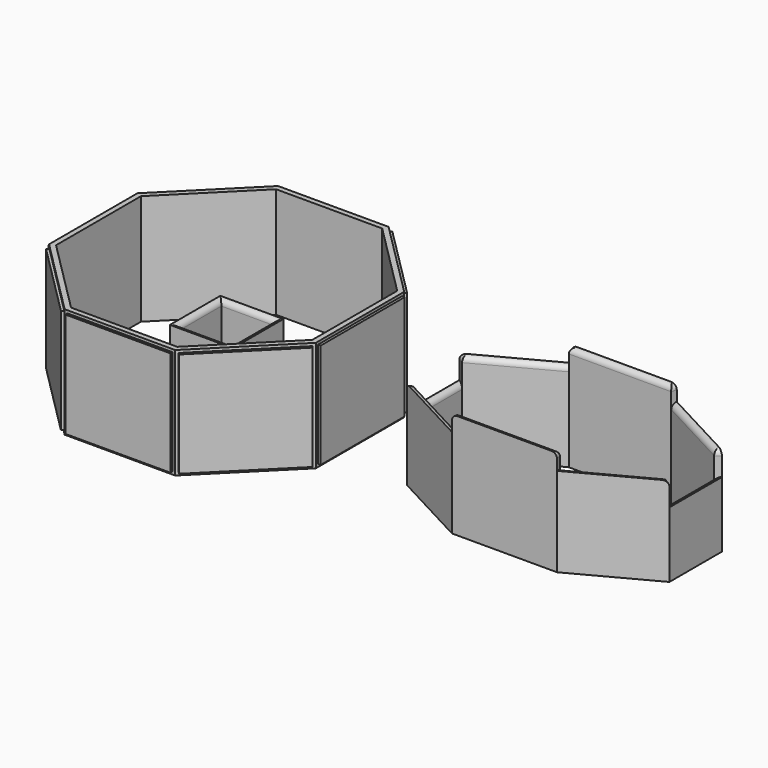
from build123d import *

# Parameters (mm, degrees)
F1_DEPTH  = 42.0840916
F2_W      = 24
F2_H      = 24
F2_W_2    = 20
F2_H_2    = 20
F3_DEPTH  = 24
F4_W      = 40
F4_H      = 40
F5_DEPTH  = 1
F7_COUNT  = 8
F9_DEPTH  = 25
F10_DEPTH = 40
F11_DEPTH = 34
F12_R     = 1.99999
F13_R     = 1.99999


# Not quite as in the source:
# - a fillet or chamfer is up to 0.001 mm smaller than in the source, because OpenCascade refuses the exact size


with BuildPart() as f1:
    # F0 (on Top) → F1 (new body)
    with BuildSketch(Plane.XY):
        Polygon((-50.8, 21.0420489686), (-50.8, -21.0420489686), (-21.0420489686, -50.8), (21.0420489686, -50.8), (50.8, -21.0420489686), (50.8, 21.0420489686), (21.0420489686, 50.8), (-21.0420489686, 50.8), align=None)
        Polygon((-20.2136218438, -48.8), (-48.8, -20.2136218438), (-48.8, 20.2136218438), (-20.2136218438, 48.8), (20.2136218438, 48.8), (48.8, 20.2136218438), (48.8, -20.2136218438), (20.2136218438, -48.8), align=None, mode=Mode.SUBTRACT)
    extrude(amount=F1_DEPTH)


with BuildPart() as f3:
    # F2 (on Top) → F3 (new body)
    with BuildSketch(Plane.XY):
        Rectangle(F2_W, F2_H)
        Rectangle(F2_W_2, F2_H_2, mode=Mode.SUBTRACT)
    extrude(amount=F3_DEPTH)

    # F13 (radius 2 in the source; OpenCascade refuses exactly that, so slightly less here)
    f13_edges = [f3.edges().sort_by_distance(p)[0] for p in [
        (0, 10, 24),
        (-10, 0, 24),
        (10, 0, 24),
        (0, -10, 24),
    ]]
    fillet(f13_edges, radius=F13_R)


with BuildPart() as f5:
    # F4 (on face) → F5 (new body, symmetric)
    with BuildSketch(Plane(origin=(0, 50.8, 0), x_dir=(-1, 0, 0), z_dir=(0, 1, 0))):
        with Locations((0, 21.0420458)):
            Rectangle(F4_W, F4_H)
    extrude(amount=F5_DEPTH, both=True)


with BuildPart() as f7_1:
    # F7: instance of F5
    add(f5.part.rotate(Axis((0, 0, 32.1497656405), (0, 0, 1)), 1 * 360 / F7_COUNT))


with BuildPart() as f7_2:
    # F7: instance of F5
    add(f5.part.rotate(Axis((0, 0, 32.1497656405), (0, 0, 1)), 2 * 360 / F7_COUNT))


with BuildPart() as f7_3:
    # F7: instance of F5
    add(f5.part.rotate(Axis((0, 0, 32.1497656405), (0, 0, 1)), 3 * 360 / F7_COUNT))


with BuildPart() as f7_4:
    # F7: instance of F5
    add(f5.part.rotate(Axis((0, 0, 32.1497656405), (0, 0, 1)), 4 * 360 / F7_COUNT))


with BuildPart() as f7_5:
    # F7: instance of F5
    add(f5.part.rotate(Axis((0, 0, 32.1497656405), (0, 0, 1)), 5 * 360 / F7_COUNT))


with BuildPart() as f7_6:
    # F7: instance of F5
    add(f5.part.rotate(Axis((0, 0, 32.1497656405), (0, 0, 1)), 6 * 360 / F7_COUNT))


with BuildPart() as f7_7:
    # F7: instance of F5
    add(f5.part.rotate(Axis((0, 0, 32.1497656405), (0, 0, 1)), 7 * 360 / F7_COUNT))


with BuildPart() as f9:
    # F8 (on Top) → F9 (new body)
    with BuildSketch(Plane.XY):
        Polygon((78.6284790199, 12.5), (78.6284790199, 0), (78.6284790199, -12.5), (80.6284790199, -11.3), (80.6284790199, 0), (80.6284790199, 11.3), align=None)
    extrude(amount=F9_DEPTH)



with BuildPart() as f9b:
    # F8 (on Top) → F9, piece 2 (new body)
    with BuildSketch(Plane.XY):
        Polygon((178.6284790199, 0), (178.6284790199, 12.5), (176.6284790199, 11.3), (176.6284790199, 0), (176.6284790199, -11.3), (178.6284790199, -12.5), align=None)
    extrude(amount=F9_DEPTH)


with BuildPart() as f10:
    # F8 (on Top) → F10 (new body)
    with BuildSketch(Plane.XY):
        Polygon((148.6284790199, 28.5), (108.6284790199, 28.5), (109.1284790199, 26.5), (148.1284790199, 26.5), align=None)
    extrude(amount=F10_DEPTH)


with BuildPart() as f10b:
    # F8 (on Top) → F10, piece 2 (new body)
    with BuildSketch(Plane.XY):
        Polygon((109.1284790199, -26.5), (108.6284790199, -28.5), (148.6284790199, -28.5), (148.1284790199, -26.5), align=None)
    extrude(amount=F10_DEPTH)


with BuildPart() as f9_1:
    add(f9.part)

    add(f9b.part)  # F11 merges F9b

    add(f10.part)  # F11 merges F10

    add(f10b.part)  # F11 merges F10b
    # F8 (on Top) → F11 (join)
    with BuildSketch(Plane.XY):
        Polygon((148.1284790199, -26.5), (148.6284790199, -28.5), (178.6284790199, -12.5), (176.6284790199, -11.3), align=None)
        Polygon((80.6284790199, -11.3), (78.6284790199, -12.5), (108.6284790199, -28.5), (109.1284790199, -26.5), align=None)
        Polygon((108.6284790199, 28.5), (78.6284790199, 12.5), (80.6284790199, 11.3), (109.1284790199, 26.5), align=None)
        Polygon((178.6284790199, 12.5), (148.6284790199, 28.5), (148.1284790199, 26.5), (176.6284790199, 11.3), align=None)
    extrude(amount=F11_DEPTH)

    # F12 (radius 2 in the source; OpenCascade refuses exactly that, so slightly less here)
    f12_edges = [f9_1.edges().sort_by_distance(p)[0] for p in [
        (80.628479, 0, 25),
        (94.878479, -18.9, 34),
        (128.628479, 26.5, 40),
        (162.378479, 18.9, 34),
        (176.628479, 0, 25),
        (162.378479, -18.9, 34),
        (128.628479, -26.5, 40),
        (94.878479, 18.9, 34),
        (79.628479, 11.9, 34),
        (108.878479, 27.5, 40),
        (148.378479, 27.5, 40),
        (177.628479, 11.9, 34),
        (177.628479, -11.9, 34),
        (148.378479, -27.5, 40),
        (108.878479, -27.5, 40),
        (79.628479, -11.9, 34),
    ]]
    fillet(f12_edges, radius=F12_R)


solid = Compound([f1.part, f3.part, f5.part, f7_1.part, f7_2.part, f7_3.part, f7_4.part, f7_5.part, f7_6.part, f7_7.part, f9_1.part])
